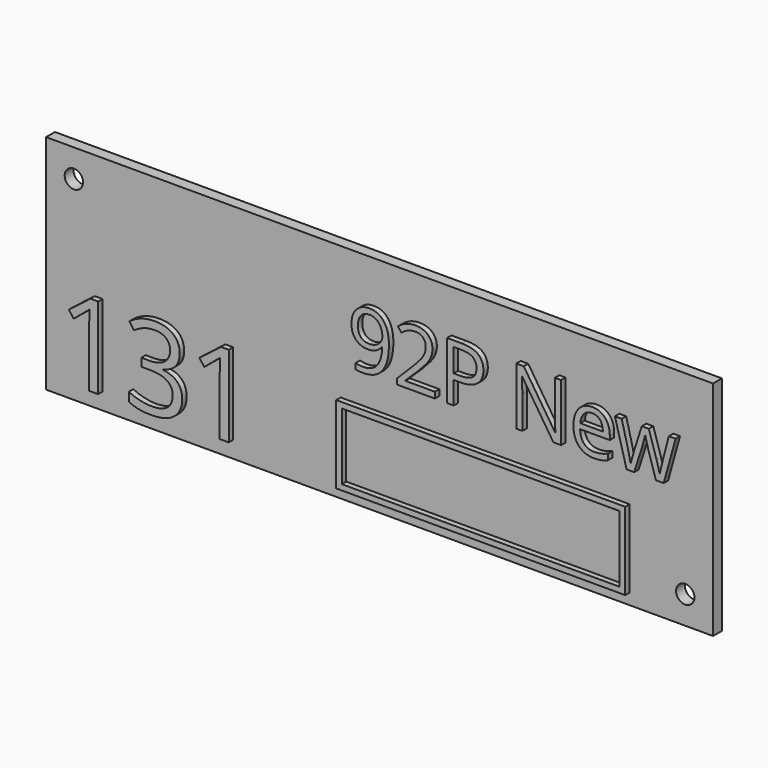
from build123d import *

# Parameters (mm, degrees)
F0_W         = 120
F0_H         = 40
F1_DEPTH     = 2
F3_D         = 3.3
F4_TEXT_SIZE = 14.4502144954
F5_DEPTH     = 1
F6_TEXT_SIZE = 20.5478077656
F7_DEPTH     = 1
F8_W         = 52
F8_H         = 14
F8_W_2       = 49.99999962
F8_H_2       = 11.99999962
F9_DEPTH     = 1


# Not quite as in the source:
# - Text() gives the source's letters only with a copy of the font that has no kerning and outlines rounded to 1/6400 em; it was checked with that copy


with BuildPart() as f1:
    # F0 (on Front) → F1 (new body)
    with BuildSketch(Plane.XZ):
        Rectangle(F0_W, F0_H)
    extrude(amount=F1_DEPTH)

    # F3 (through all)
    with Locations(Plane.XZ.offset(2)):
        with Locations((-55, 15), (55, -15)):
            Hole(F3_D / 2)

    # F4 (on face) → F5 (join)
    with BuildSketch(Plane.XZ.offset(2)):
        with Locations((-5, 2)):
            Text('92P New', F4_TEXT_SIZE, font='Open Sans', text_align=(TextAlign.LEFT, TextAlign.BOTTOM))
    extrude(amount=F5_DEPTH)

    # F6 (on face) → F7 (join)
    with BuildSketch(Plane.XZ.offset(2)):
        with Locations((-57, -17)):
            Text('131', F6_TEXT_SIZE, font='Open Sans', text_align=(TextAlign.LEFT, TextAlign.BOTTOM))
    extrude(amount=F7_DEPTH)

    # F8 (on face) → F9 (join)
    with BuildSketch(Plane.XZ.offset(2)):
        with Locations((19, -11)):
            Rectangle(F8_W, F8_H)
        with Locations((19, -11)):
            Rectangle(F8_W_2, F8_H_2, mode=Mode.SUBTRACT)
    extrude(amount=F9_DEPTH)


solid = f1.part
